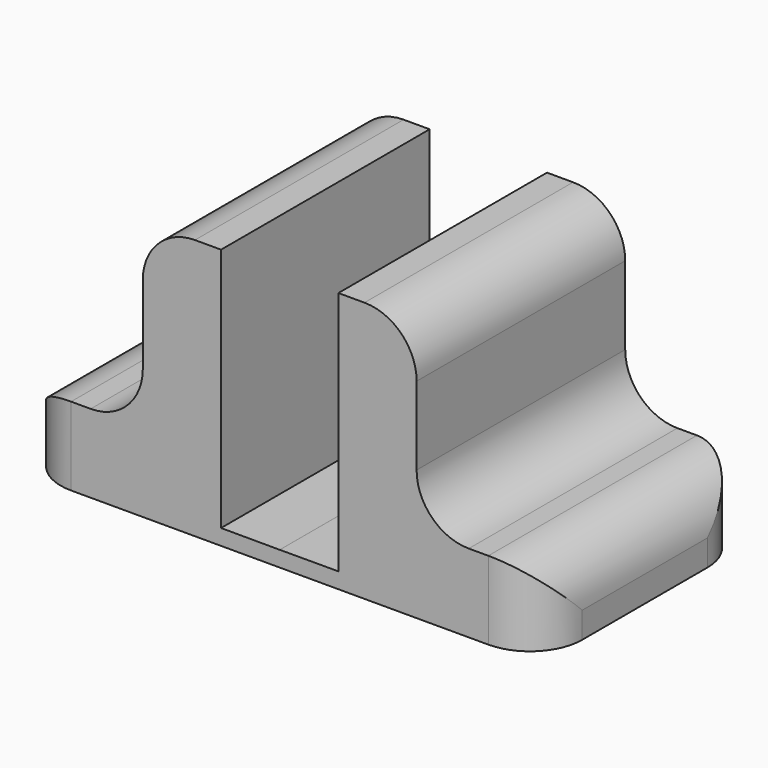
from build123d import *

# Parameters (mm, degrees)
F1_DEPTH = 10
F2_R     = 2


# Not quite as in the source:
# - ends of sketch curves that miss each other by under 0.0002 mm in the source are joined


with BuildPart() as f1:
    # F0 (on Front) → F1 (new body)
    with BuildSketch(Plane.XZ):
        Polygon((-0.0010415313, 0.600002712), (-2.25, 0.6039066758), (-2.25, 10), (-5.25, 10), (-5.25, 3), (-10, 3), (-10, 0), (0, 0), align=None)
        Polygon((0.0010415376, 0.599999096), (-0.0010415313, 0.600002712), (0, 0), align=None)
        Polygon((2.25, 0.6039066758), (0.0010415313, 0.600002712), (0, 0), (10, 0), (10, 3), (5.25, 3), (5.25, 10), (2.25, 10), align=None)
    extrude(amount=F1_DEPTH)

    # F2
    f2_edges = [f1.edges().sort_by_distance(p)[0] for p in [
        (-5.25, -5, 3),
        (5.25, -5, 3),
        (10, -5, 3),
        (5.25, -5, 10),
        (-5.25, -5, 10),
        (-10, -5, 3),
        (-10, -10, 1.5),
        (-10, 0, 1.5),
        (10, -10, 1.5),
        (10, 0, 1.5),
    ]]
    fillet(f2_edges, radius=F2_R)


solid = f1.part
